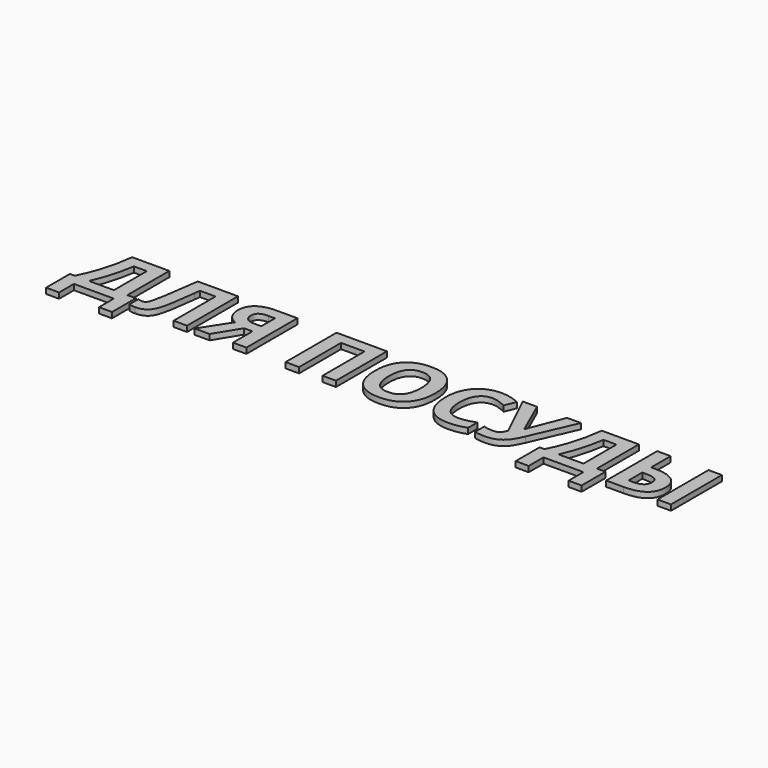
from build123d import *

# Parameters (mm, degrees)
F0_TEXT_SIZE = 15.9182381405
F1_DEPTH     = 1


# Not quite as in the source:
# - Text() gives the source's letters only with a copy of the font that has no kerning and outlines rounded to 1/6400 em; it was checked with that copy


with BuildPart() as f1:
    # F0 (on Top) → F1 (new body)
    with BuildSketch(Plane.XY):
        with Locations((0, -11.4611314611)):
            Text('ДЛЯ ПОСУДЫ', F0_TEXT_SIZE, font='Open Sans', font_style=FontStyle.BOLD, text_align=(TextAlign.LEFT, TextAlign.BOTTOM))
    extrude(amount=F1_DEPTH)


solid = f1.part
